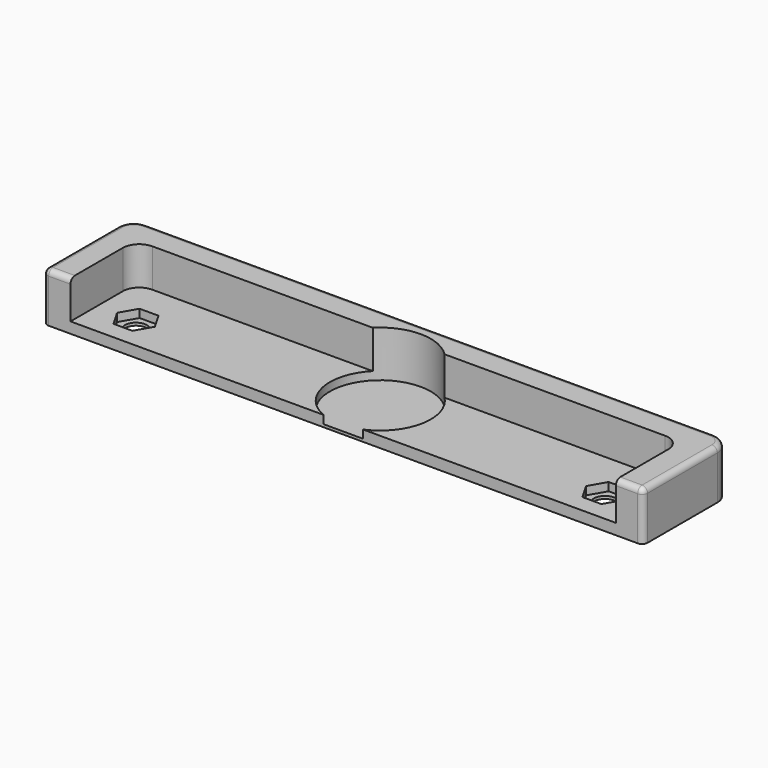
from build123d import *

# Parameters (mm, degrees)
F0_W           = 110
F0_H           = 20
F1_DEPTH       = 9
F2_W           = 100
F2_H           = 15
F3_DEPTH       = 7
F4_R           = 3
F5_R           = 2
F6_DEPTH       = 20
F8_DEPTH       = 1.5
F9_R           = 9.25
F10_DEPTH      = 1.5
F10_DEPTH_BACK = 7
F11_R          = 1


with BuildPart() as f1:
    # F0 (on Top) → F1 (new body)
    with BuildSketch(Plane.XY):
        with Locations((6.7567551136, -16.7820947109)):
            Rectangle(F0_W, F0_H)
    extrude(amount=F1_DEPTH)

    # F2 (on face) → F3 (cut)
    with BuildSketch(Plane.XY.offset(9)):
        with Locations((6.7567551136, -19.2820947109)):
            Rectangle(F2_W, F2_H)
    extrude(amount=-F3_DEPTH, mode=Mode.SUBTRACT)

    # F4
    f4_edges = [f1.edges().sort_by_distance(p)[0] for p in [
        (-43.243245, -11.782095, 5.5),
        (56.756755, -11.782095, 5.5),
        (-48.243245, -6.782095, 4.5),
        (61.756755, -6.782095, 4.5),
    ]]
    fillet(f4_edges, radius=F4_R)

    # F5 (on face) → F6 (cut)
    with BuildSketch(Plane.XY.offset(2)):
        with Locations((49.7567551136, -20.5320947109)):
            Circle(F5_R)
        with Locations((-36.2432448864, -20.5320947109)):
            Circle(F5_R)
    extrude(amount=-F6_DEPTH, mode=Mode.SUBTRACT)

    # F7 (on face) → F8 (cut)
    with BuildSketch(Plane.XY.offset(2)):
        Polygon((-34.5111940788, -17.5320947109), (-37.975295694, -17.5320947109), (-39.7073465015, -20.5320947109), (-37.975295694, -23.5320947109), (-34.5111940788, -23.5320947109), (-32.7791432713, -20.5320947109), align=None)
        Polygon((53.2208567287, -20.5320947109), (51.4888059212, -17.5320947109), (48.024704306, -17.5320947109), (46.2926534985, -20.5320947109), (48.024704306, -23.5320947109), (51.4888059212, -23.5320947109), align=None)
    extrude(amount=-F8_DEPTH, mode=Mode.SUBTRACT)

    # F9 (on face) → F10 (cut, two sides)
    with BuildSketch(Plane.XY.offset(2)) as f10_sk:
        with Locations((6.7567551136, -18.2820947109)):
            Circle(F9_R)
    extrude(amount=-F10_DEPTH, mode=Mode.SUBTRACT)
    extrude(f10_sk.sketch, amount=F10_DEPTH_BACK, mode=Mode.SUBTRACT)

    # F11
    f11_edges = [f1.edges().sort_by_distance(p)[0] for p in [
        (6.756755, -6.782095, 9),
        (-48.243245, -26.782095, 4.5),
        (61.756755, -26.782095, 4.5),
        (59.256755, -26.782095, 9),
        (-45.743245, -26.782095, 9),
    ]]
    fillet(f11_edges, radius=F11_R)


solid = f1.part
